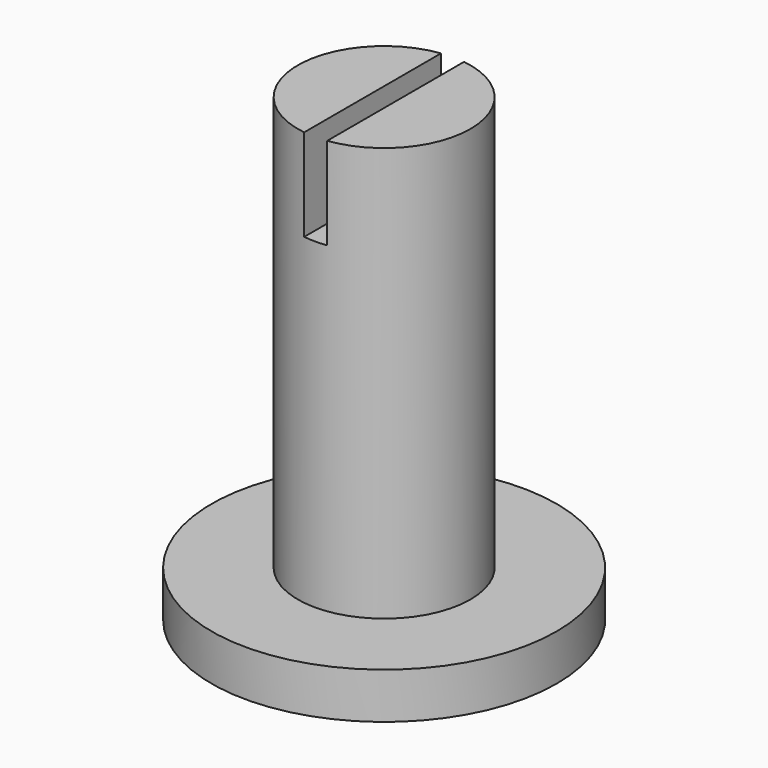
from build123d import *

# Parameters (mm, degrees)
F0_R     = 1.875
F1_DEPTH = 10
F0_R_2   = 3.75
F2_DEPTH = 1
F4_DEPTH = 2


with BuildPart() as f1:
    # F0 (on Top) → F1 (new body)
    with BuildSketch(Plane.XY):
        Circle(F0_R)
    extrude(amount=F1_DEPTH)

    # F0 (on Top) → F2 (join)
    with BuildSketch(Plane.XY):
        Circle(F0_R_2)
        Circle(F0_R, mode=Mode.SUBTRACT)
    extrude(amount=F2_DEPTH)

    # F3 (on face) → F4 (cut)
    with BuildSketch(Plane.XY.offset(10)):
        with BuildLine():
            Line((-0.25, 1.8582585934), (-0.25, -1.8582585934))
            ThreePointArc((-0.25, -1.8582585934), (0, -1.875), (0.25, -1.8582585934))
            Line((0.25, -1.8582585934), (0.25, 1.8582585934))
            ThreePointArc((0.25, 1.8582585934), (0, 1.875), (-0.25, 1.8582585934))
        make_face()
        with BuildLine():
            Line((-0.25, 2.5), (-0.25, 1.8582585934))
            ThreePointArc((-0.25, 1.8582585934), (0, 1.875), (0.25, 1.8582585934))
            Line((0.25, 1.8582585934), (0.25, 2.5))
            Line((0.25, 2.5), (-0.25, 2.5))
        make_face()
    extrude(amount=-F4_DEPTH, mode=Mode.SUBTRACT)


solid = f1.part
